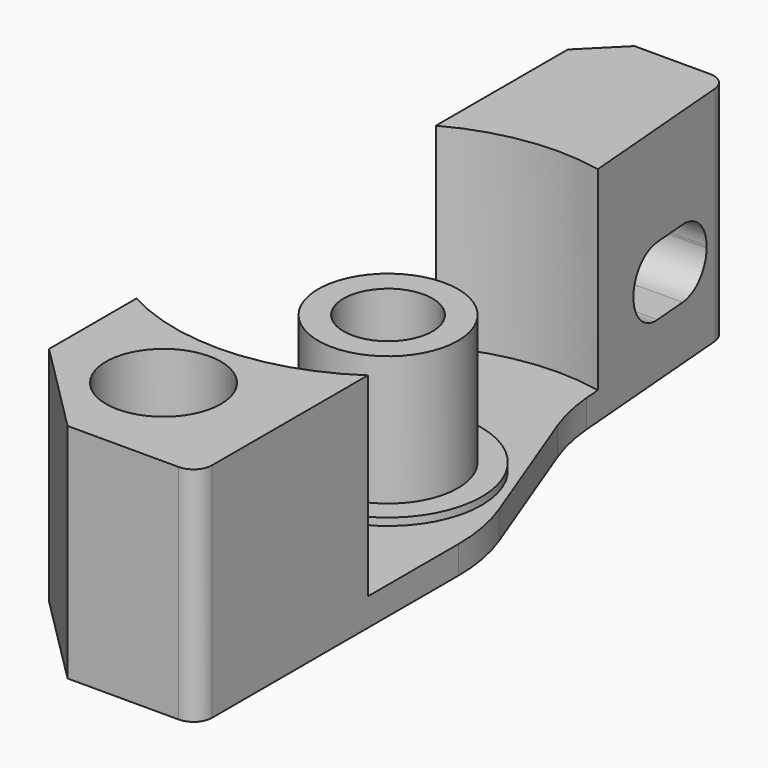
from build123d import *

# Parameters (mm, degrees)
F1_W            = 12
F1_H            = 42
F2_DEPTH        = 12
F7_R            = 11.5
F7_R_2          = 3.775
F9_DEPTH        = 25
F8_R            = 5.05
F10_DEPTH       = 0.4
F11_D           = 4.8
F12_D           = 3.5
F12_CBORE_D     = 6.2
F12_CBORE_DEPTH = 9
F14_DEPTH       = 25
F16_DEPTH       = 25
F17_SIZE        = 5
F18_T1_DEPTH    = 22.2867319519
F19_R           = 1
F20_R           = 4.5
F21_DEPTH       = 3.1
F22_R           = 10


# Not quite as in the source:
# - a fillet or chamfer that OpenCascade refuses, or shapes differently, is made with other operations: its cross-section is extruded or revolved along the edge and cut away or added


with BuildPart() as f2:
    # F1 (on Top) → F2 (new body)
    with BuildSketch(Plane.XY):
        with Locations((-6, 21)):
            Rectangle(F1_W, F1_H)
    extrude(amount=F2_DEPTH)

    # F7 (on offset) → F9 (cut)
    with BuildSketch(Plane.XY.offset(1.5)):
        with Locations((-6.5, 21)):
            Circle(F7_R)
        with Locations((-6.5, 21)):
            Circle(F7_R_2, mode=Mode.SUBTRACT)
    extrude(amount=F9_DEPTH, mode=Mode.SUBTRACT)

    # F8 (on offset) → F10 (join)
    with BuildSketch(Plane.XY.offset(1.5)):
        with Locations((-6.5, 21)):
            Circle(F8_R)
    extrude(amount=F10_DEPTH)

    # F11 (through all)
    with Locations(Plane(origin=(0, 0, 0), x_dir=(1, 0, 0), z_dir=(0, 0, -1))):
        with Locations((-6.5, -21)):
            Hole(F11_D / 2)

    # F12 (through all)
    with Locations(Plane.XY.offset(12)):
        with Locations((-6.3, 5.6)):
            CounterBoreHole(F12_D / 2, F12_CBORE_D / 2, F12_CBORE_DEPTH)

    # F13 (on Top) → F14 (cut)
    with BuildSketch(Plane.XY):
        Polygon((-5, 42), (-4, 30), (0, 19.4664706794), (0, 42), align=None)
    extrude(amount=F14_DEPTH, mode=Mode.SUBTRACT)

    # F15 (on offset) → F16 (cut)
    with BuildSketch(Plane(origin=(-12, 0, 0), x_dir=(0, -1, 0), z_dir=(-1, 0, 0))):
        with BuildLine():
            Line((-36.75, 6.6), (-38.65, 6.6))
            ThreePointArc((-38.65, 6.6), (-39.9227922061, 6.0727922061), (-40.45, 4.8))
            Line((-40.45, 4.8), (-40.45, 4.7))
            ThreePointArc((-40.45, 4.7), (-39.9227922061, 3.4272077939), (-38.65, 2.9))
            Line((-38.65, 2.9), (-36.75, 2.9))
            ThreePointArc((-36.75, 2.9), (-35.4772077939, 3.4272077939), (-34.95, 4.7))
            Line((-34.95, 4.7), (-34.95, 4.8))
            ThreePointArc((-34.95, 4.8), (-35.4772077939, 6.0727922061), (-36.75, 6.6))
        make_face()
    extrude(amount=-F16_DEPTH, mode=Mode.SUBTRACT)

    # F17
    f17_edges = [f2.edges().sort_by_distance(p)[0] for p in [
        (-12, 0, 6),
    ]]
    chamfer(f17_edges, length=F17_SIZE)

    # F18: chamfer of 2 on 1 edges, made by hand

    # F18_s2 → F18_t1 (cut)
    with BuildSketch(Plane.XY.offset(-5.1433659759)):
        Polygon((-12, 40), (-10, 42), (-12, 42), align=None)
    extrude(amount=F18_T1_DEPTH, mode=Mode.SUBTRACT)

    # F19
    f19_edges = [f2.edges().sort_by_distance(p)[0] for p in [
        (0, 0, 6),
        (-5, 42, 6),
    ]]
    fillet(f19_edges, radius=F19_R)

    # F20 (on offset) → F21 (cut)
    with BuildSketch(Plane.XY.offset(12)):
        with Locations((-6.5, 21)):
            Circle(F20_R)
    extrude(amount=-F21_DEPTH, mode=Mode.SUBTRACT)

    # F22
    f22_edges = [f2.edges().sort_by_distance(p)[0] for p in [
        (-4, 30, 0.75),
        (0, 19.466471, 0.75),
    ]]
    fillet(f22_edges, radius=F22_R)


solid = f2.part
